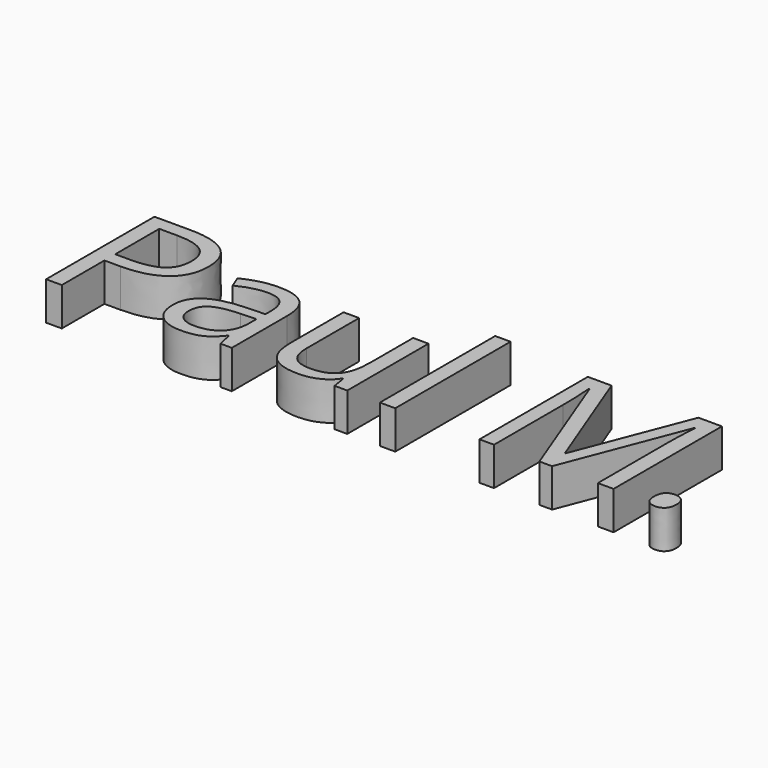
from build123d import *

# Parameters (mm, degrees)
F0_TEXT_SIZE = 12.4000711647
F1_DEPTH     = 2.5


# Not quite as in the source:
# - Text() gives the source's letters only with a copy of the font that has no kerning and outlines rounded to 1/6400 em; it was checked with that copy


with BuildPart() as f1:
    # F0 (on Top) → F1 (new body)
    with BuildSketch(Plane.XY):
        with Locations((-42.7085576068, -8.9280512386)):
            Text('Paul M.', F0_TEXT_SIZE, font='Open Sans', text_align=(TextAlign.LEFT, TextAlign.BOTTOM))
    extrude(amount=F1_DEPTH)


solid = f1.part
